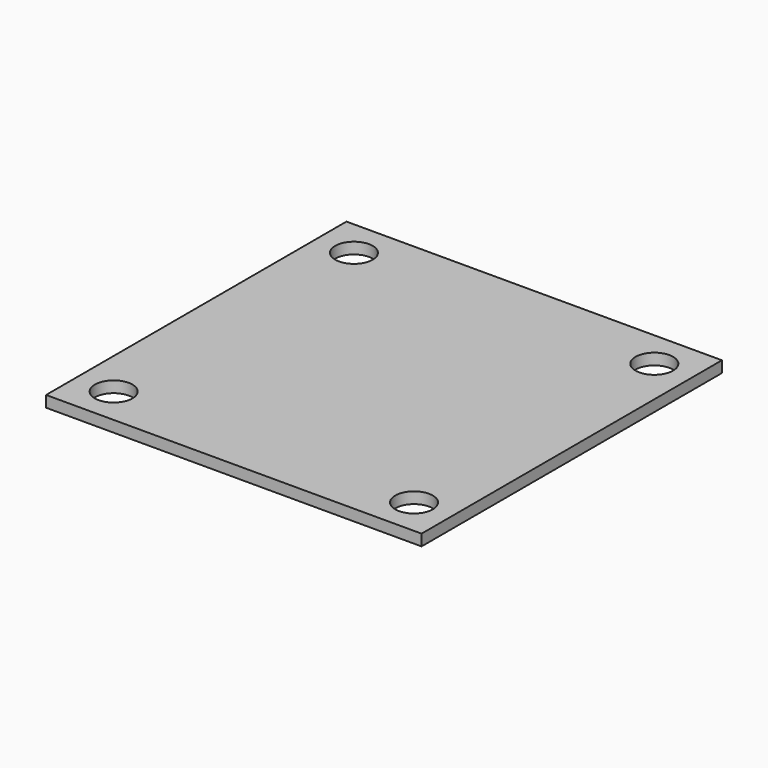
from build123d import *

# Parameters (mm, degrees)
F0_W     = 100
F0_H     = 100
F1_DEPTH = 3
F2_R     = 5
F3_DEPTH = 25


# Not quite as in the source:
# - the program builds the solid bodies; features that only make, move or delete a surface that nothing else refers to are left out


with BuildPart() as f1:
    # F0 (on Top) → F1 (new body)
    with BuildSketch(Plane.XY):
        Rectangle(F0_W, F0_H)
    extrude(amount=F1_DEPTH)

    # F2 (on face) → F3 (cut)
    with BuildSketch(Plane(origin=(0, 0, 0), x_dir=(1, 0, 0), z_dir=(0, 0, -1))):
        with Locations((40, 40)):
            Circle(F2_R)
        with Locations((40, -40)):
            Circle(F2_R)
        with Locations((-40, -40)):
            Circle(F2_R)
        with Locations((-40, 40)):
            Circle(F2_R)
    extrude(amount=-F3_DEPTH, mode=Mode.SUBTRACT)


solid = f1.part
